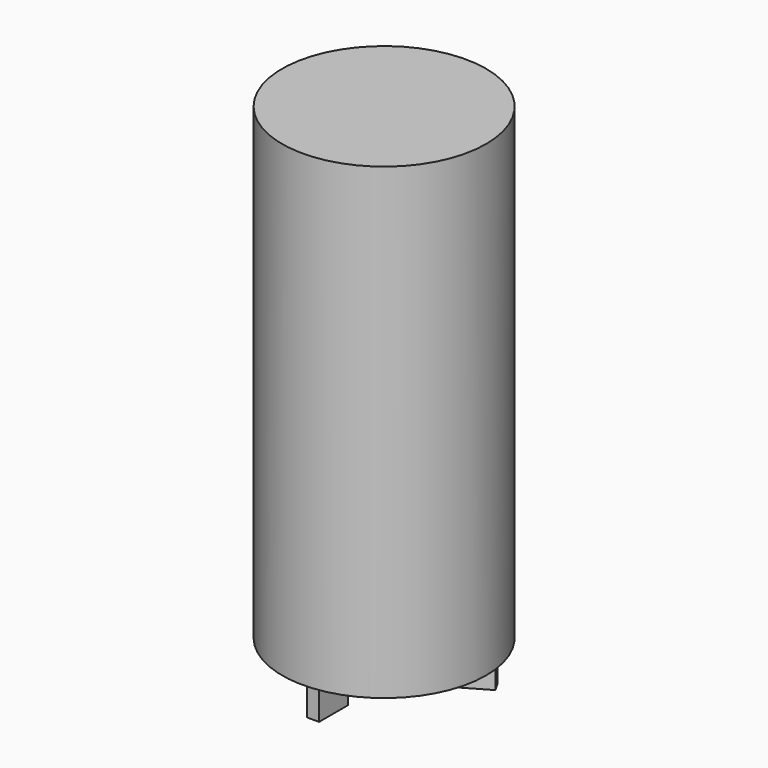
from build123d import *

# Parameters (mm, degrees)
F0_R            = 425
F1_DEPTH        = 1950
F2_W            = 50
F2_H            = 150
F3_DEPTH        = 150
F3_COPIES_COUNT = 3


# Not quite as in the source:
# - a pattern or mirror of a feature is missing from the dataset's text; its kind, count and spacing are read off the source's solid


with BuildPart() as f1:
    # F0 (on Top) → F1 (new body)
    with BuildSketch(Plane.XY):
        Circle(F0_R)
    extrude(amount=F1_DEPTH)

    # F2 (on face) → F3 (join)
    with BuildSketch(Plane(origin=(0, 0, 0), x_dir=(1, 0, 0), z_dir=(0, 0, -1))):
        with Locations((0, 295)):
            Rectangle(F2_W, F2_H)
    f3 = extrude(amount=F3_DEPTH)

    # F3_copies: F3 ×3 about axis
    f3_copies_axis = Axis((0, 0, 0), (0, 0, 1))
    for i in range(1, F3_COPIES_COUNT):
        add(f3.rotate(f3_copies_axis, i * 360 / F3_COPIES_COUNT))


solid = f1.part
